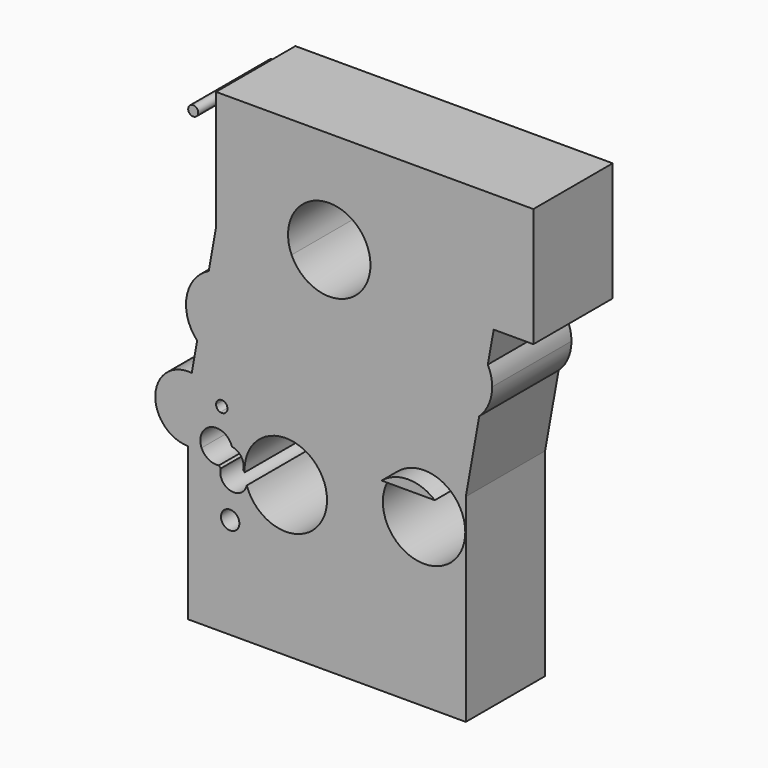
from build123d import *

# Parameters (mm, degrees)
F1_DEPTH = 25
F2_DEPTH = 30
F0_R     = 2.3197134373
F3_DEPTH = 25
F0_R_2   = 1.2608238745


with BuildPart() as f1:
    # F0 (on Front) → F1 (new body)
    with BuildSketch(Plane.XZ):
        with BuildLine():
            Line((-36.8970455988, -1.3415312964), (-38.2563615468, -8.9548247595))
            ThreePointArc((-38.2563615468, -8.9548247595), (-34.5600498563, -10.2898813947), (-31.8921704478, -13.1756249373))
            ThreePointArc((-31.8921704478, -13.1756249373), (-30.2780449791, -12.5680611078), (-29.2430992407, -13.9477067703))
            Line((-29.2430992407, -13.9477067703), (13.6264225575, -13.9477067703))
            ThreePointArc((13.6264225575, -13.9477067703), (20.327998141, -11.4977905039), (27.0295737244, -13.9477067703))
            Line((27.0295737244, -13.9477067703), (30.8521840286, -13.9477067703))
            Line((30.8521840286, -13.9477067703), (34.2387321722, 5.0197635093))
            ThreePointArc((34.2387321722, 5.0197635093), (16.8699466245, 14.3954719517), (36.4101090954, 17.1812700081))
            Line((36.4101090954, 17.1812700081), (37.8828033788, 25.4295759134))
            Line((37.8828033788, 25.4295759134), (5.9121937531, 25.4295759134))
            ThreePointArc((5.9121937531, 25.4295759134), (-3.5799022512, 19.265938237), (-13.0719982556, 25.4295759134))
            Line((-13.0719982556, 25.4295759134), (-32.1171966212, 25.4295759134))
            Line((-32.1171966212, 25.4295759134), (-33.9708996127, 15.0473061488))
            ThreePointArc((-33.9708996127, 15.0473061488), (-23.8546677668, 14.6023681954), (-18.9206845351, 5.7597483341))
            ThreePointArc((-18.9206845351, 5.7597483341), (-25.4938465616, -3.9043311549), (-36.8970455988, -1.3415312964))
        make_face()
        with BuildLine():
            ThreePointArc((27.0295737244, -13.9477067703), (20.327998141, -11.4977905039), (13.6264225575, -13.9477067703))
            Line((13.6264225575, -13.9477067703), (27.0295737244, -13.9477067703))
        make_face()
    extrude(amount=F1_DEPTH)

    # F0 (on Front) → F2 (join)
    with BuildSketch(Plane.XZ):
        with BuildLine():
            ThreePointArc((27.0295737244, -13.9477067703), (20.327998141, -11.4977905039), (13.6264225575, -13.9477067703))
            Line((13.6264225575, -13.9477067703), (27.0295737244, -13.9477067703))
        make_face()
    extrude(amount=F2_DEPTH)

    # F0 (on Front) → F3 (join)
    with BuildSketch(Plane.XZ):
        with BuildLine():
            Line((-38.2563615468, -8.9548247595), (-39.1478159714, -13.9477067703))
            Line((-39.1478159714, -13.9477067703), (-32.1171966212, -13.9477067703))
            ThreePointArc((-32.1171966212, -13.9477067703), (-32.0597935936, -13.5456038184), (-31.8921704478, -13.1756249373))
            ThreePointArc((-31.8921704478, -13.1756249373), (-34.5600498563, -10.2898813947), (-38.2563615468, -8.9548247595))
        make_face()
        with BuildLine():
            Line((-32.1171966212, -13.9477067703), (-39.1478159714, -13.9477067703))
            Line((-39.1478159714, -13.9477067703), (-39.1478159714, -25.5079631141))
            ThreePointArc((-39.1478159714, -25.5079631141), (-37.4242994609, -25.3270577869), (-35.7759086803, -24.7922272215))
            ThreePointArc((-35.7759086803, -24.7922272215), (-35.1346869248, -20.5881831631), (-31.1005712876, -19.2424258261))
            ThreePointArc((-31.1005712876, -19.2424258261), (-30.9108182069, -18.2327612754), (-30.8472425547, -17.2073896974))
            ThreePointArc((-30.8472425547, -17.2073896974), (-30.9010050472, -16.2641884324), (-31.0615960895, -15.3332053234))
            ThreePointArc((-31.0615960895, -15.3332053234), (-31.8232289681, -14.8186112891), (-32.1171966212, -13.9477067703))
        make_face()
        with BuildLine():
            Line((-39.1478159714, -25.5079631141), (-39.1478159714, -13.9477067703))
            Line((-39.1478159714, -13.9477067703), (-38.2563615468, -8.9548247595))
            ThreePointArc((-38.2563615468, -8.9548247595), (-47.4363785787, -16.7610165897), (-39.1478159714, -25.5079631141))
        make_face()
        with BuildLine():
            ThreePointArc((-35.7759086803, -24.7922272215), (-37.4242994609, -25.3270577869), (-39.1478159714, -25.5079631141))
            Line((-39.1478159714, -25.5079631141), (-39.1478159714, -63.9477067703))
            Line((-39.1478159714, -63.9477067703), (30.8521840286, -63.9477067703))
            Line((30.8521840286, -63.9477067703), (30.8521840286, -13.9477067703))
            Line((30.8521840286, -13.9477067703), (27.0295737244, -13.9477067703))
            ThreePointArc((27.0295737244, -13.9477067703), (29.7514687642, -17.510578657), (30.71880327, -21.8885956329))
            ThreePointArc((30.71880327, -21.8885956329), (15.949981165, -31.3120662561), (13.6264225575, -13.9477067703))
            Line((13.6264225575, -13.9477067703), (-29.2430992407, -13.9477067703))
            ThreePointArc((-29.2430992407, -13.9477067703), (-29.8092434122, -15.0907878075), (-31.0615960895, -15.3332053234))
            ThreePointArc((-31.0615960895, -15.3332053234), (-30.9010050472, -16.2641884324), (-30.8472425547, -17.2073896974))
            ThreePointArc((-30.8472425547, -17.2073896974), (-30.9108182069, -18.2327612754), (-31.1005712876, -19.2424258261))
            ThreePointArc((-31.1005712876, -19.2424258261), (-29.2348911506, -20.2350073875), (-28.1168713895, -22.0283317708))
            ThreePointArc((-28.1168713895, -22.0283317708), (-26.0187057491, -23.153295251), (-25.1810509111, -25.3817871757))
            ThreePointArc((-25.1810509111, -25.3817871757), (-25.209190214, -25.817226894), (-25.2931400278, -26.2454231077))
            ThreePointArc((-25.2931400278, -26.2454231077), (-25.0909422893, -26.4646669846), (-24.908839255, -26.7008666627))
            ThreePointArc((-24.908839255, -26.7008666627), (-14.8376440321, -15.7106090516), (-4.1447894931, -26.0970231288))
            ThreePointArc((-4.1447894931, -26.0970231288), (-12.8539883778, -36.3508532263), (-24.3821109254, -29.4159006375))
            ThreePointArc((-24.3821109254, -29.4159006375), (-28.4932406364, -31.9295574903), (-30.9476780862, -27.7828003139))
            ThreePointArc((-30.9476780862, -27.7828003139), (-31.1826286879, -27.5241383485), (-31.3896450432, -27.2426209845))
            ThreePointArc((-31.3896450432, -27.2426209845), (-34.0051544965, -26.7734902048), (-35.7759086803, -24.7922272215))
        make_face()
        with Locations((-28.5642116289, -38.4677797556)):
            Circle(F0_R, mode=Mode.SUBTRACT)
        with BuildLine():
            Line((-36.8970455988, -1.3415312964), (-38.2563615468, -8.9548247595))
            ThreePointArc((-38.2563615468, -8.9548247595), (-34.5600498563, -10.2898813947), (-31.8921704478, -13.1756249373))
            ThreePointArc((-31.8921704478, -13.1756249373), (-30.2780449791, -12.5680611078), (-29.2430992407, -13.9477067703))
            Line((-29.2430992407, -13.9477067703), (13.6264225575, -13.9477067703))
            ThreePointArc((13.6264225575, -13.9477067703), (20.327998141, -11.4977905039), (27.0295737244, -13.9477067703))
            Line((27.0295737244, -13.9477067703), (30.8521840286, -13.9477067703))
            Line((30.8521840286, -13.9477067703), (34.2387321722, 5.0197635093))
            ThreePointArc((34.2387321722, 5.0197635093), (16.8699466245, 14.3954719517), (36.4101090954, 17.1812700081))
            Line((36.4101090954, 17.1812700081), (37.8828033788, 25.4295759134))
            Line((37.8828033788, 25.4295759134), (5.9121937531, 25.4295759134))
            ThreePointArc((5.9121937531, 25.4295759134), (-3.5799022512, 19.265938237), (-13.0719982556, 25.4295759134))
            Line((-13.0719982556, 25.4295759134), (-32.1171966212, 25.4295759134))
            Line((-32.1171966212, 25.4295759134), (-33.9708996127, 15.0473061488))
            ThreePointArc((-33.9708996127, 15.0473061488), (-23.8546677668, 14.6023681954), (-18.9206845351, 5.7597483341))
            ThreePointArc((-18.9206845351, 5.7597483341), (-25.4938465616, -3.9043311549), (-36.8970455988, -1.3415312964))
        make_face()
        with BuildLine():
            ThreePointArc((-33.9708996127, 15.0473061488), (-39.540531436, 7.5860932242), (-36.8970455988, -1.3415312964))
            Line((-36.8970455988, -1.3415312964), (-33.9708996127, 15.0473061488))
        make_face()
        with BuildLine():
            Line((-33.9708996127, 15.0473061488), (-36.8970455988, -1.3415312964))
            ThreePointArc((-36.8970455988, -1.3415312964), (-25.4938465616, -3.9043311549), (-18.9206845351, 5.7597483341))
            ThreePointArc((-18.9206845351, 5.7597483341), (-23.8546677668, 14.6023681954), (-33.9708996127, 15.0473061488))
        make_face()
        with BuildLine():
            Line((-32.1171966212, 55.4295759134), (-32.1171966212, 25.4295759134))
            Line((-32.1171966212, 25.4295759134), (-13.0719982556, 25.4295759134))
            ThreePointArc((-13.0719982556, 25.4295759134), (-5.740725171, 39.8203881619), (6.8109028777, 29.6567433659))
            ThreePointArc((6.8109028777, 29.6567433659), (6.5837425447, 27.4959204462), (5.9121937531, 25.4295759134))
            Line((5.9121937531, 25.4295759134), (37.8828033788, 25.4295759134))
            Line((37.8828033788, 25.4295759134), (47.8828033788, 25.4295759134))
            Line((47.8828033788, 25.4295759134), (47.8828033788, 55.4295759134))
            Line((47.8828033788, 55.4295759134), (-32.1171966212, 55.4295759134))
        make_face()
        with BuildLine():
            ThreePointArc((36.4101090954, 17.1812700081), (16.8699466245, 14.3954719517), (34.2387321722, 5.0197635093))
            Line((34.2387321722, 5.0197635093), (36.4101090954, 17.1812700081))
        make_face()
        with BuildLine():
            Line((36.4101090954, 17.1812700081), (34.2387321722, 5.0197635093))
            ThreePointArc((34.2387321722, 5.0197635093), (36.6424814014, 8.4593128941), (37.4897935254, 12.5691270616))
            ThreePointArc((37.4897935254, 12.5691270616), (37.2162724179, 14.9375432533), (36.4101090954, 17.1812700081))
        make_face()
    extrude(amount=F3_DEPTH)


with BuildPart() as f3:
    # F0 (on Front) → F3, piece 2 (new body)
    with BuildSketch(Plane.XZ):
        with Locations((-37.8869920969, 49.3332110345)):
            Circle(F0_R_2)
    extrude(amount=F3_DEPTH)


solid = Compound([f1.part, f3.part])
